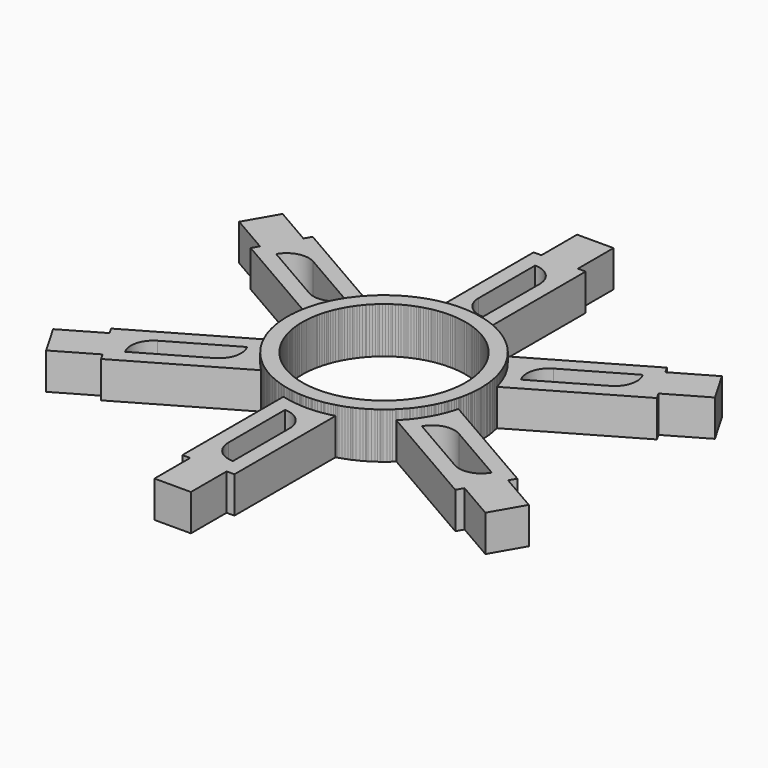
from build123d import *

# Parameters (mm, degrees)
F1_DEPTH = 6.2
F0_W     = 4.9
F0_H     = 6
F2_DEPTH = 4.9
F3_COUNT = 6


with BuildPart() as f1:
    # F0 (on Top) → F1 (new body)
    with BuildSketch(Plane.XY):
        with BuildLine():
            ThreePointArc((-3.5, 12.5199840255), (-12.8794369507, -1.7663815652), (0, -13))
            ThreePointArc((0, -13), (9.1923881554, -9.1923881554), (13, 0))
            ThreePointArc((13, 0), (10.3561575886, 7.8581168228), (3.5, 12.5199840255))
            ThreePointArc((3.5, 12.5199840255), (0, 13), (-3.5, 12.5199840255))
        make_face()
        with BuildLine():
            ThreePointArc((0, -11), (-7.7781745931, 7.7781745931), (11, 0))
            ThreePointArc((11, 0), (7.7781745931, -7.7781745931), (0, -11))
        make_face(mode=Mode.SUBTRACT)
    extrude(amount=F1_DEPTH)

    # F0 (on Top) → F2 (join)
    with BuildSketch(Plane.XY):
        with BuildLine():
            Line((-3.5, 29.5199840255), (-3.5, 12.5199840255))
            ThreePointArc((-3.5, 12.5199840255), (0, 13), (3.5, 12.5199840255))
            Line((3.5, 12.5199840255), (3.5, 29.5199840255))
            Line((3.5, 29.5199840255), (2.45, 29.5199840255))
            Line((2.45, 29.5199840255), (-2.45, 29.5199840255))
            Line((-2.45, 29.5199840255), (-3.5, 29.5199840255))
        make_face()
        with BuildLine():
            Line((1.5, 24.2727840255), (1.5, 14.7699840255))
            Line((1.5, 14.7699840255), (1.4972, 14.7699840255))
            ThreePointArc((1.4972, 14.7699840255), (-0.6221404446, 15.647843581), (-1.5, 17.7671840255))
            Line((-1.5, 17.7671840255), (-1.5, 27.2699840255))
            Line((-1.5, 27.2699840255), (-1.4972, 27.2699840255))
            ThreePointArc((-1.4972, 27.2699840255), (0.6221404446, 26.3921244701), (1.5, 24.2727840255))
        make_face(mode=Mode.SUBTRACT)
        with Locations((0, 32.5199840255)):
            Rectangle(F0_W, F0_H)
    extrude(amount=F2_DEPTH)


with BuildPart() as f3_1:
    # F3: instance of F1
    add(f1.part.rotate(Axis((0, 0, 6.2), (0, 0, 1)), 1 * 360 / F3_COUNT))


with BuildPart() as f3_2:
    # F3: instance of F1
    add(f1.part.rotate(Axis((0, 0, 6.2), (0, 0, 1)), 2 * 360 / F3_COUNT))


with BuildPart() as f3_3:
    # F3: instance of F1
    add(f1.part.rotate(Axis((0, 0, 6.2), (0, 0, 1)), 3 * 360 / F3_COUNT))


with BuildPart() as f3_4:
    # F3: instance of F1
    add(f1.part.rotate(Axis((0, 0, 6.2), (0, 0, 1)), 4 * 360 / F3_COUNT))


with BuildPart() as f3_5:
    # F3: instance of F1
    add(f1.part.rotate(Axis((0, 0, 6.2), (0, 0, 1)), 5 * 360 / F3_COUNT))


solid = Compound([f1.part, f3_1.part, f3_2.part, f3_3.part, f3_4.part, f3_5.part])
